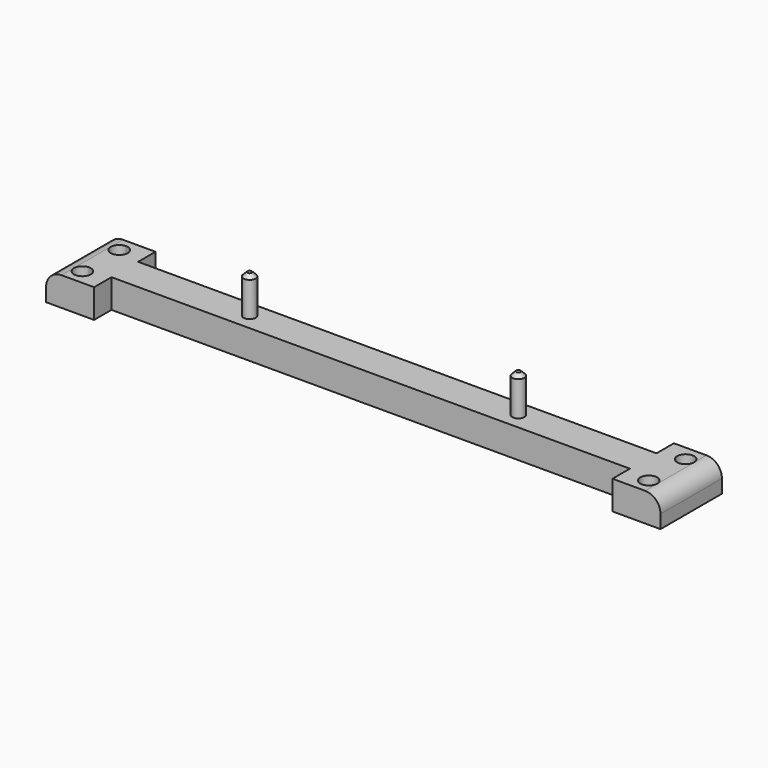
from build123d import *

# Parameters (mm, degrees)
F1_DEPTH = 9.525
F2_R     = 2.8
F3_DEPTH = 9.525
F4_R     = 2
F5_DEPTH = 12.7
F6_SIZE  = 1.27
F7_R     = 5.08
F8_R     = 2.8
F8_R_2   = 1.6
F9_DEPTH = 5


# Not quite as in the source:
# - a length typed as a fraction of an inch, garbled in the dataset ("3 / 203.2 mm" for 3/8 in), is restored


with BuildPart() as f1:
    # F0 (on Top) → F1 (new body)
    with BuildSketch(Plane.XY):
        Polygon((-85.725, -5.5000017), (85.725, -5.5000017), (85.725, -12.7), (101.6, -12.7), (101.6, -5.5000017), (101.6, 5.5000017), (101.6, 12.7), (85.725, 12.7), (85.725, 5.5000017), (-85.725, 5.5000017), (-85.725, 12.7), (-101.6, 12.7), (-101.6, 5.5000017), (-101.6, -5.5000017), (-101.6, -12.7), (-85.725, -12.7), align=None)
    extrude(amount=F1_DEPTH)

    # F2 (on face) → F3 (cut, through all)
    with BuildSketch(Plane.XY.offset(9.525)):
        with BuildLine():
            ThreePointArc((-93.6625, 4.82), (-91.6826010127, 5.6401010127), (-90.8625, 7.62))
            ThreePointArc((-90.8625, 7.62), (-91.6826010127, 9.5998989873), (-93.6625, 10.42))
            Line((-93.6625, 10.42), (-93.6625, 4.82))
        make_face()
        with BuildLine():
            ThreePointArc((-90.8625, -7.62), (-91.6826010127, -5.6401010127), (-93.6625, -4.82))
            Line((-93.6625, -4.82), (-93.6625, -10.42))
            ThreePointArc((-93.6625, -10.42), (-91.6826010127, -9.5998989873), (-90.8625, -7.62))
        make_face()
        with BuildLine():
            Line((-93.6625, -10.42), (-93.6625, -4.82))
            ThreePointArc((-93.6625, -4.82), (-96.4625, -7.62), (-93.6625, -10.42))
        make_face()
        with BuildLine():
            Line((-93.6625, 4.82), (-93.6625, 10.42))
            ThreePointArc((-93.6625, 10.42), (-96.4625, 7.62), (-93.6625, 4.82))
        make_face()
        with Locations((93.6625, 7.62)):
            Circle(F2_R)
        with Locations((93.6625, -7.62)):
            Circle(F2_R)
    extrude(amount=-F3_DEPTH, mode=Mode.SUBTRACT)

    # F4 (on face) → F5 (join)
    with BuildSketch(Plane.XY.offset(9.525)):
        with Locations((-44.45, 0)):
            Circle(F4_R)
        with Locations((44.45, 0)):
            Circle(F4_R)
    extrude(amount=F5_DEPTH)

    # F6
    f6_edges = [f1.edges().sort_by_distance(p)[0] for p in [
        (-46.45, 0, 22.225),
        (42.45, 0, 22.225),
    ]]
    chamfer(f6_edges, length=F6_SIZE)

    # F7
    f7_edges = [f1.edges().sort_by_distance(p)[0] for p in [
        (-101.6, 0, 9.525),
        (101.6, 0, 9.525),
    ]]
    fillet(f7_edges, radius=F7_R)

    # F8 (on face) → F9 (join)
    with BuildSketch(Plane(origin=(0, 0, 0), x_dir=(1, 0, 0), z_dir=(0, 0, -1))):
        with Locations((93.6625, 7.62)):
            Circle(F8_R)
        with Locations((93.6625, 7.62)):
            Circle(F8_R_2, mode=Mode.SUBTRACT)
        with Locations((93.6625, -7.62)):
            Circle(F8_R)
        with Locations((93.6625, -7.62)):
            Circle(F8_R_2, mode=Mode.SUBTRACT)
        with Locations((-93.6625, 7.62)):
            Circle(F8_R)
        with Locations((-93.6625, 7.62)):
            Circle(F8_R_2, mode=Mode.SUBTRACT)
        with Locations((-93.6625, -7.62)):
            Circle(F8_R)
        with Locations((-93.6625, -7.62)):
            Circle(F8_R_2, mode=Mode.SUBTRACT)
    extrude(amount=-F9_DEPTH)


solid = f1.part
